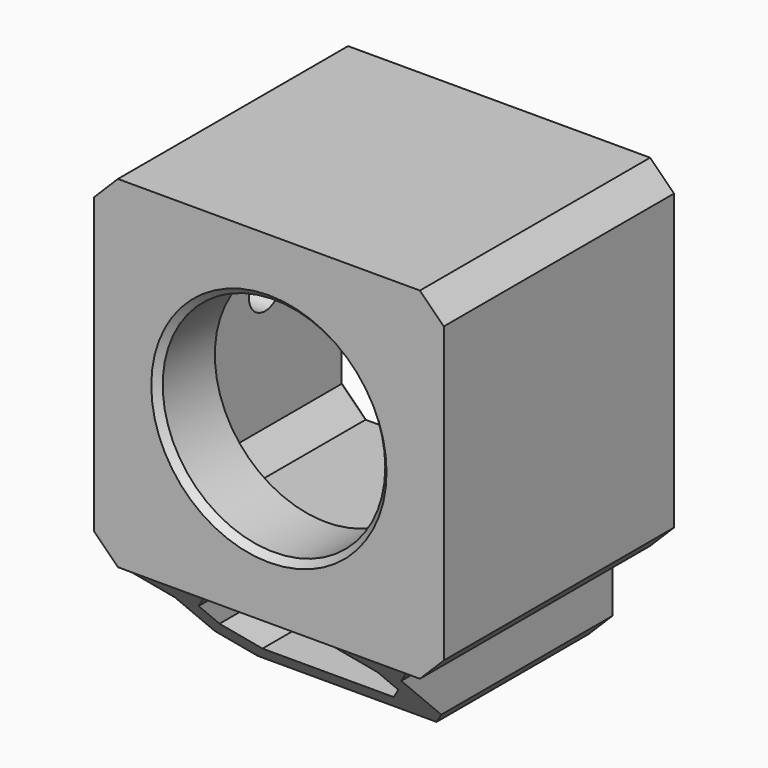
from build123d import *

# Parameters (mm, degrees)
F0_W        = 44
F0_H        = 43
F0_W_2      = 38
F0_H_2      = 37
F1_DEPTH    = 27.2
F2_W        = 44
F2_H        = 43
F2_R        = 14
F3_DEPTH    = 9
F4_SIZE     = 3
F6_DEPTH    = 36.2
F7_SIZE     = 3
F8_T1_DEPTH = 85.763401504
F9_R        = 2.55
F10_DEPTH   = 3
F11_SIZE    = 0.8
F12_SIZE    = 1


# Not quite as in the source:
# - a fillet or chamfer that OpenCascade refuses, or shapes differently, is made with other operations: its cross-section is extruded or revolved along the edge and cut away or added


with BuildPart() as f1:
    # F0 (on Front) → F1 (new body)
    with BuildSketch(Plane.XZ):
        Rectangle(F0_W, F0_H)
        Rectangle(F0_W_2, F0_H_2, mode=Mode.SUBTRACT)
    extrude(amount=F1_DEPTH)

    # F2 (on face) → F3 (join)
    with BuildSketch(Plane.XZ.offset(27.2)):
        Rectangle(F2_W, F2_H)
        Circle(F2_R, mode=Mode.SUBTRACT)
    extrude(amount=F3_DEPTH)

    # F4
    f4_edges = [f1.edges().sort_by_distance(p)[0] for p in [
        (22, -18.1, 21.5),
        (22, -18.1, -21.5),
        (-22, -18.1, -21.5),
        (-22, -18.1, 21.5),
        (-19, -13.6, 18.5),
        (-19, -13.6, -18.5),
        (19, -13.6, -18.5),
        (19, -13.6, 18.5),
    ]]
    chamfer(f4_edges, length=F4_SIZE)

    # F5 (on face) → F6 (join, through all)
    with BuildSketch(Plane.XZ.offset(36.2)):
        Polygon((-14.25, -33.8), (14.25, -33.8), (14.25, -21.5), (11.25, -21.5), (11.25, -30.8), (-11.25, -30.8), (-11.25, -21.5), (-14.25, -21.5), align=None)
    extrude(amount=-F6_DEPTH)

    # F7
    f7_edges = [f1.edges().sort_by_distance(p)[0] for p in [
        (-14.25, -18.1, -33.8),
        (-14.25, -18.1, -21.5),
        (-11.25, -18.1, -30.8),
        (11.25, -18.1, -30.8),
        (11.25, -18.1, -21.5),
        (14.25, -18.1, -33.8),
        (14.25, -18.1, -21.5),
        (-11.25, -18.1, -21.5),
    ]]
    chamfer(f7_edges, length=F7_SIZE)

    # F8: chamfer of 12.3 on 1 edges, made by hand

    # F8_s2 → F8_t1 (cut)
    with BuildSketch(Plane.YZ.offset(-42.881700752)):
        Polygon((-36.2, -21.5), (-23.9, -33.8), (-36.2, -33.8), align=None)
    extrude(amount=F8_T1_DEPTH, mode=Mode.SUBTRACT)

    # F9 (on face) → F10 (cut, through all)
    with BuildSketch(Plane(origin=(-22, 0, 0), x_dir=(0, -1, 0), z_dir=(-1, 0, 0))):
        with Locations((13.05, 0)):
            Circle(F9_R)
    extrude(amount=-F10_DEPTH, mode=Mode.SUBTRACT)

    # F11
    f11_edges = [f1.edges().sort_by_distance(p)[0] for p in [
        (-14, -36.2, 0),
    ]]
    chamfer(f11_edges, length=F11_SIZE)

    # F12
    f12_edges = [f1.edges().sort_by_distance(p)[0] for p in [
        (0, 0, 18.5),
        (19, 0, 0),
        (0, 0, -18.5),
        (-19, 0, 0),
        (17.5, 0, 17),
        (17.5, 0, -17),
        (-17.5, 0, -17),
        (-17.5, 0, 17),
    ]]
    chamfer(f12_edges, length=F12_SIZE)


solid = f1.part
